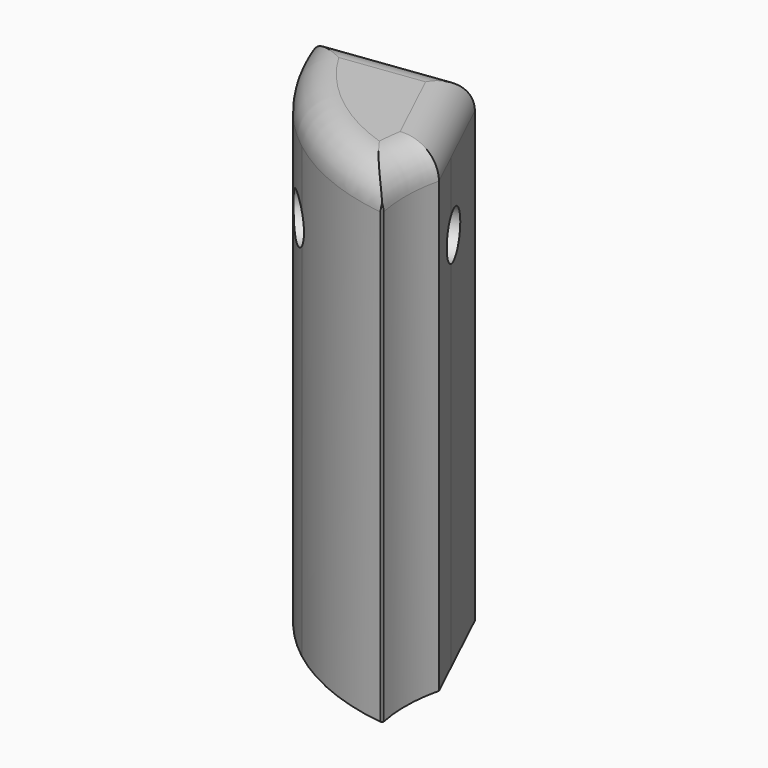
from build123d import *

# Parameters (mm, degrees)
F1_DEPTH    = 25.4
F2_T1_DEPTH = 15.3225079539
F2_T3_DEPTH = 16.775320589
F2_T6_ANGLE = 87.0348581142
F2_T8_ANGLE = 103.9234369613
F3_R        = 1.2082658068
F4_DEPTH    = 25.4


# Not quite as in the source:
# - a fillet or chamfer that OpenCascade refuses, or shapes differently, is made with other operations: its cross-section is extruded or revolved along the edge and cut away or added


with BuildPart() as f1:
    # F0 (on Top) → F1 (new body)
    with BuildSketch(Plane.XY):
        with BuildLine():
            ThreePointArc((-7.752480221, -10.059276834), (-4.8810304794, -8.8387254095), (-2.3312001475, -7.0405778413))
            Line((-2.3312001475, -7.0405778413), (-4.1826744651, -3.1376440612))
            Line((-4.1826744651, -3.1376440612), (-12.0026959047, -4.1503362537))
            ThreePointArc((-12.0026959047, -4.1503362537), (-10.3099777223, -7.4158181858), (-7.752480221, -10.059276834))
        make_face()
        with BuildLine():
            ThreePointArc((-1.4857464298, -12.5192106342), (-1.6518399037, -10.7309962936), (-1.4257026774, -8.9493791841))
            Line((-1.4257026774, -8.9493791841), (-2.3312001475, -7.0405778413))
            ThreePointArc((-2.3312001475, -7.0405778413), (-4.8810304794, -8.8387254095), (-7.752480221, -10.059276834))
            ThreePointArc((-7.752480221, -10.059276834), (-4.8332265428, -11.7443569933), (-1.5735123086, -12.6021450164))
            Line((-1.5735123086, -12.6021450164), (-1.4857464298, -12.5192106342))
        make_face()
    extrude(amount=F1_DEPTH)

    # F2: fillet of radius 1.778 on 4 edges, made by hand

    # F2_s2 → F2_t1 (cut)
    with BuildSketch(Plane(origin=(5.1087634899, -10.7693449534, 0), x_dir=(0, 0, 1), z_dir=(-0.4285998257, 0.9034944324, 0))):
        with BuildLine():
            ThreePointArc((23.622, -5.1238167896), (24.8792358569, -5.6445809326), (25.4, -6.9018167896))
            Line((25.4, -6.9018167896), (25.4, -5.1238167896))
            Line((25.4, -5.1238167896), (23.622, -5.1238167896))
        make_face()
    extrude(amount=F2_T1_DEPTH, mode=Mode.SUBTRACT)

    # F2_s4 → F2_t3 (cut)
    with BuildSketch(Plane(origin=(-0.1051193903, -0.0136129532, 0), x_dir=(0, 0, 1), z_dir=(-0.9917188973, -0.1284275232, 0))):
        with BuildLine():
            ThreePointArc((23.622, -2.5744903868), (24.8792358569, -3.0952545299), (25.4, -4.3524903868))
            Line((25.4, -4.3524903868), (25.4, -2.5744903868))
            Line((25.4, -2.5744903868), (23.622, -2.5744903868))
        make_face()
    extrude(amount=F2_T3_DEPTH, mode=Mode.SUBTRACT)

    # F2_s5 → F2_t6 (revolve, cut)
    with BuildSketch(Plane(origin=(8.4191230763, -9.1705520677, 0), x_dir=(0, 0, 1), z_dir=(0.6762824344, -0.7366424295, 0))):
        with BuildLine():
            ThreePointArc((23.622, 10.7336378697), (24.8792358569, 11.2544020127), (25.4, 12.5116378697))
            Line((25.4, 12.5116378697), (25.4, 10.7336378697))
            Line((25.4, 10.7336378697), (23.622, 10.7336378697))
        make_face()
    revolve(axis=Axis((6.5687949782, -10.8692655012, 25.4), (0, 0, -1)), revolution_arc=F2_T6_ANGLE, mode=Mode.SUBTRACT)

    # F2_s7 → F2_t8 (revolve, cut)
    with BuildSketch(Plane(origin=(0, 0, 0), x_dir=(0, 0, 1), z_dir=(0.017156123, 0.9998528229, 0))):
        with BuildLine():
            ThreePointArc((23.622, -12.7), (24.8792358569, -12.1792358569), (25.4, -10.922))
            Line((25.4, -10.922), (25.4, -12.7))
            Line((25.4, -12.7), (23.622, -12.7))
        make_face()
    revolve(axis=Axis((0, 0, 25.4), (0, 0, 1)), revolution_arc=F2_T8_ANGLE, mode=Mode.SUBTRACT)

    # F3 (on face) → F4 (cut)
    with BuildSketch(Plane(origin=(-4.6293399422, -2.1960669829, 0), x_dir=(-0.4285998257, 0.9034944324, 0), z_dir=(0.9034944324, 0.4285998257, 0))):
        with Locations((-4.8675471917, 19.804911688)):
            Circle(F3_R)
    extrude(amount=-F4_DEPTH, mode=Mode.SUBTRACT)


solid = f1.part
